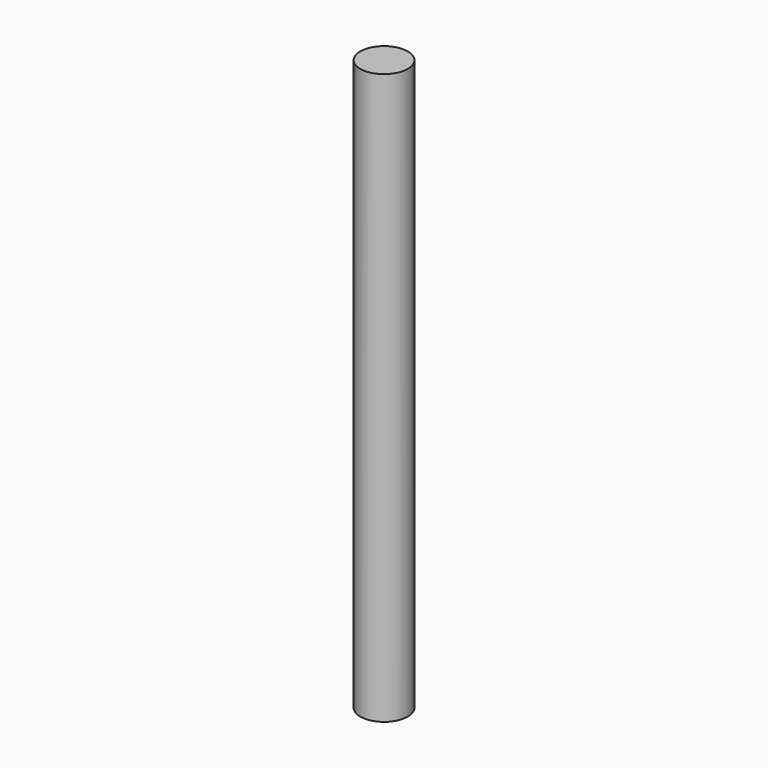
from build123d import *

# Parameters (mm, degrees)
F1_R     = 6.35
F2_DEPTH = 152.4


# Not quite as in the source:
# - a variable given as a bare number and used for a length is read in inches; the dataset says mm whatever the document's units were


with BuildPart() as f2:
    # F1 (on Top) → F2 (new body)
    with BuildSketch(Plane.XY):
        Circle(F1_R)
    extrude(amount=F2_DEPTH)


solid = f2.part
